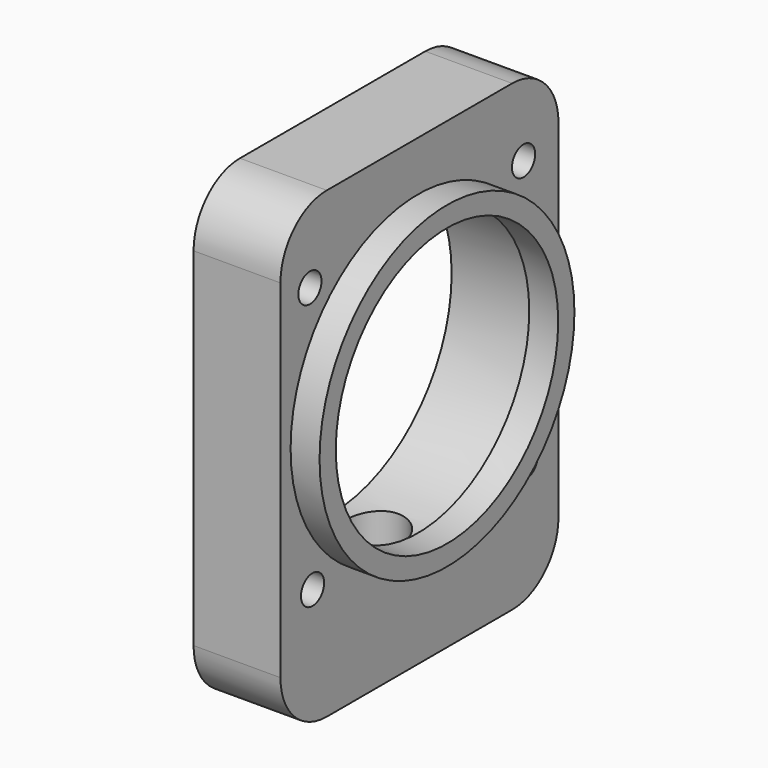
from build123d import *

# Parameters (mm, degrees)
F0_R     = 6.985
F0_R_2   = 6.096
F1_DEPTH = 1.27
F2_R     = 6.604
F3_DEPTH = 3.81
F5_D     = 1.27
F7_D     = 2.54
F7_DEPTH = 5.08
F7_TIP   = 0.7630929862


# Not quite as in the source:
# - a feature names something its author has since deleted; it is built from what else it names


with BuildPart() as f1:
    # F0 (on Right) → F1 (new body)
    with BuildSketch(Plane.YZ):
        Circle(F0_R)
        Circle(F0_R_2, mode=Mode.SUBTRACT)
    extrude(amount=F1_DEPTH)

    # F2 (on Right) → F3 (join)
    with BuildSketch(Plane.YZ):
        with BuildLine():
            Line((5.1588201895, 9.1668736476), (-5.0011798105, 9.1668736476))
            ThreePointArc((-5.0011798105, 9.1668736476), (-6.7972310347, 8.4229248718), (-7.5411798105, 6.6268736476))
            Line((-7.5411798105, 6.6268736476), (-7.5411798105, -8.6131263524))
            ThreePointArc((-7.5411798105, -8.6131263524), (-6.7972310347, -10.4091775766), (-5.0011798105, -11.1531263524))
            Line((-5.0011798105, -11.1531263524), (5.1588201895, -11.1531263524))
            ThreePointArc((5.1588201895, -11.1531263524), (6.9548714137, -10.4091775766), (7.6988201895, -8.6131263524))
            Line((7.6988201895, -8.6131263524), (7.6988201895, 6.6268736476))
            ThreePointArc((7.6988201895, 6.6268736476), (6.9548714137, 8.4229248718), (5.1588201895, 9.1668736476))
        make_face()
        Circle(F2_R, mode=Mode.SUBTRACT)
    extrude(amount=-F3_DEPTH)

    # F5 (through all)
    with Locations(Plane(origin=(-3.81, 0, 0), x_dir=(0, -1, 0), z_dir=(-1, 0, 0))):
        with Locations((5.9254106074, 5.7839893926), (-5.7839893926, 5.9254106074), (5.7839893926, -5.9254106074), (-5.9254106074, -5.7839893926)):
            Hole(F5_D / 2)

    # F7
    with Locations(Plane(origin=(0, 0, -11.1531263524), x_dir=(1, 0, 0), z_dir=(0, 0, -1))):
        with Locations((-1.8845667364, 0)):
            Hole(F7_D / 2, depth=F7_DEPTH)
            with Locations((0, 0, -(F7_DEPTH + F7_TIP / 2))):  # 118° drill point
                Cone(0, F7_D / 2, F7_TIP, mode=Mode.SUBTRACT)


solid = f1.part
